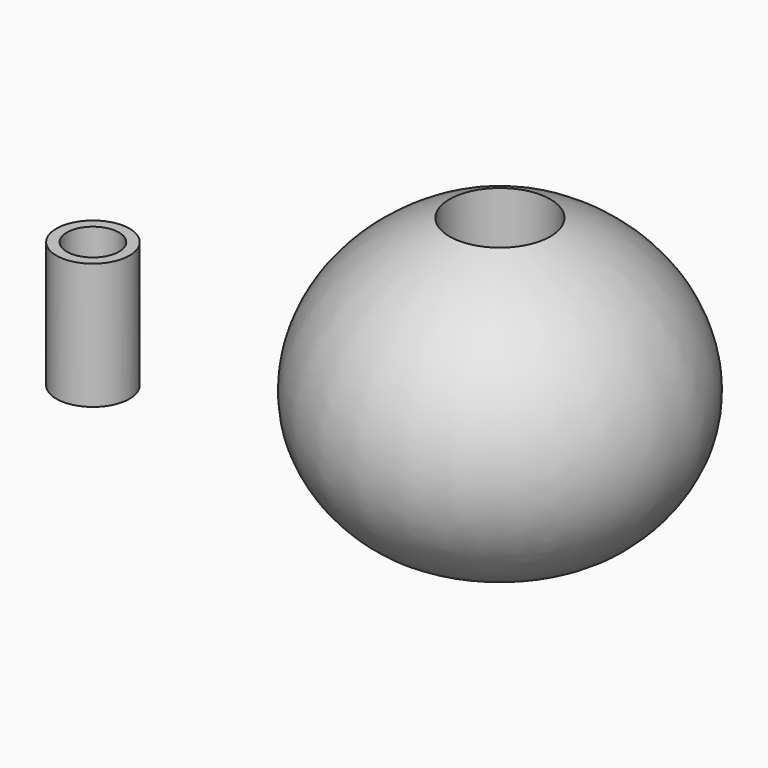
from build123d import *

# Parameters (mm, degrees)
F0_R     = 5.5245
F0_R_2   = 3.937
F1_DEPTH = 19.05


# Not quite as in the source:
# - a feature names something its author has since deleted; it is built from what else it names


with BuildPart() as f1:
    # F0 (on Top) → F1 (new body)
    with BuildSketch(Plane.XY):
        with Locations((-115.8623099327, 6.6972491331)):
            Circle(F0_R)
        with Locations((-115.8623099327, 6.6972491331)):
            Circle(F0_R_2, mode=Mode.SUBTRACT)
    extrude(amount=F1_DEPTH)


with BuildPart() as f1_1:
    # F3: moved
    add(f1.part.moved(Location((54.3814, -6.6802, 0))))


with BuildPart() as f4:
    # F2 (on Front) → F4 (revolve)
    with BuildSketch(Plane.XZ):
        with BuildLine():
            Line((5.588, 31.115), (5.588, 13.335))
            Line((5.588, 13.335), (7.62, 13.335))
            Line((7.62, 13.335), (7.62, 0.1780921506))
            add(Edge.make_bspline(
                [(7.62, 42.2705757692), (15.0955538915, 39.4168298845), (25.5425060258, 30.5591890241), (27.5617616639, 13.6550365202), (18.1713954603, 2.2547557748), (12.3616936725, 0.4867159105), (7.62, 0.1780921506)],
                knots=[0.0724738741, 0.0724738741, 0.0724738741, 0.0724738741, 0.3058367763, 0.5402018073, 0.7535449183, 0.9251048332, 0.9251048332, 0.9251048332, 0.9251048332], degree=3))
            Line((7.62, 42.2705757692), (7.62, 31.115))
            Line((7.62, 31.115), (5.588, 31.115))
        make_face()
    revolve(axis=Axis((0, 0, 13.802273199), (0, 0, -1)))


solid = Compound([f1_1.part, f4.part])
